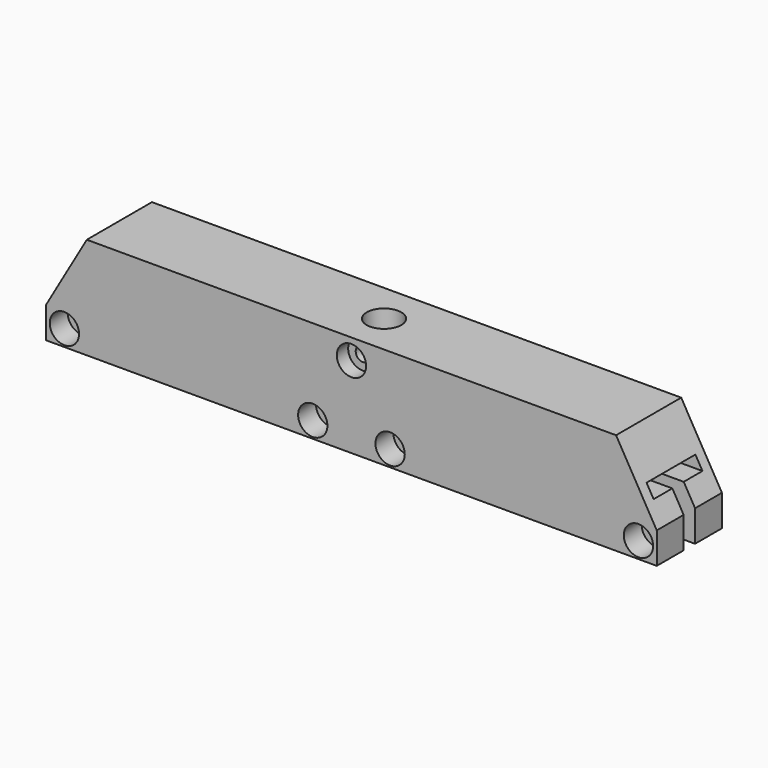
from build123d import *

# Parameters (mm, degrees)
F1_DEPTH       = 10
F3_DEPTH       = 7.5
F5_R           = 4.25
F6_DEPTH       = 30
F8_D           = 4
F8_DEPTH       = 8.5
F8_CBORE_D     = 7.2
F8_CBORE_DEPTH = 5.5
F8_TIP         = 1.2017212381
F9_D           = 3.5
F9_DEPTH       = 7
F9_CBORE_D     = 7.2
F9_CBORE_DEPTH = 3.5
F9_TIP         = 1.0515060833
F10_R          = 5
F11_R          = 5
F12_W          = 3.5
F12_H          = 12.5
F13_DEPTH      = 150.001
F7_R           = 1.1
F14_DEPTH      = 18
F15_T1_DEPTH   = 109.6192794117
F16_T1_DEPTH   = 109.6192794117


# Not quite as in the source:
# - a fillet or chamfer that OpenCascade refuses, or shapes differently, is made with other operations: its cross-section is extruded or revolved along the edge and cut away or added


with BuildPart() as f1:
    # F0 (on Front) → F1 (new body)
    with BuildSketch(Plane.XZ):
        Polygon((75, 12.5), (-75, 12.5), (-75, -12.5), (-50.5, -12.5), (75, -12.5), align=None)
    extrude(amount=-F1_DEPTH)

    # F2 (on face) → F3 (cut)
    with BuildSketch(Plane.XZ):
        with BuildLine():
            Line((-50.5, 0), (-50.5, -12.5))
            Line((-50.5, -12.5), (-29.5, -12.5))
            Line((-29.5, -12.5), (-29.5, 0))
            ThreePointArc((-29.5, 0), (-29.5018489924, 1.0611519764), (-29.616133488, 2.116133488))
            ThreePointArc((-29.616133488, 2.116133488), (-32.4157560185, 7.5842439815), (-37.883866512, 10.383866512))
            ThreePointArc((-37.883866512, 10.383866512), (-38.9388480236, 10.4981510076), (-40, 10.5))
            ThreePointArc((-40, 10.5), (-46.7951402173, 8.2937242033), (-50.383866512, 2.116133488))
            ThreePointArc((-50.383866512, 2.116133488), (-50.4981510076, 1.0611519764), (-50.5, 0))
        make_face()
        with BuildLine():
            ThreePointArc((29.616133488, 2.116133488), (29.5018489924, 1.0611519764), (29.5, 0))
            Line((29.5, 0), (29.5, -12.5))
            Line((29.5, -12.5), (50.5, -12.5))
            Line((50.5, -12.5), (50.5, 0))
            ThreePointArc((50.5, 0), (50.4981510076, 1.0611519764), (50.383866512, 2.116133488))
            ThreePointArc((50.383866512, 2.116133488), (47.5842439815, 7.5842439815), (42.116133488, 10.383866512))
            ThreePointArc((42.116133488, 10.383866512), (41.0611519764, 10.4981510076), (40, 10.5))
            ThreePointArc((40, 10.5), (38.9388480236, 10.4981510076), (37.883866512, 10.383866512))
            ThreePointArc((37.883866512, 10.383866512), (32.4157560185, 7.5842439815), (29.616133488, 2.116133488))
        make_face()
        with BuildLine():
            Line((-65, -12.5), (-59.4149563834, -12.5))
            Line((-59.4149563834, -12.5), (-50.5, -12.5))
            Line((-50.5, -12.5), (-50.5, 0))
            ThreePointArc((-50.5, 0), (-50.4981510076, 1.0611519764), (-50.383866512, 2.116133488))
            Line((-50.383866512, 2.116133488), (-65, -12.5))
        make_face()
        Polygon((-29.5, 0), (-29.5, -12.5), (-15, -12.5), (-27.5, 0), align=None)
        with BuildLine():
            ThreePointArc((-29.616133488, 2.116133488), (-29.5018489924, 1.0611519764), (-29.5, 0))
            Line((-29.5, 0), (-27.5, 0))
            Line((-27.5, 0), (-29.616133488, 2.116133488))
        make_face()
        Polygon((27.5, 0), (15, -12.5), (17, -12.5), (19.8756534234, -12.5), (29.5, -12.5), (29.5, 0), align=None)
        with BuildLine():
            Line((29.616133488, 2.116133488), (27.5, 0))
            Line((27.5, 0), (29.5, 0))
            ThreePointArc((29.5, 0), (29.5018489924, 1.0611519764), (29.616133488, 2.116133488))
        make_face()
        with BuildLine():
            Line((50.5, 0), (52.5, 0))
            Line((52.5, 0), (50.383866512, 2.116133488))
            ThreePointArc((50.383866512, 2.116133488), (50.4981510076, 1.0611519764), (50.5, 0))
        make_face()
        Polygon((62.5, -10.8300764114), (62.5, -10), (52.5, 0), (50.5, 0), (50.5, -12.5), (62.5, -12.5), align=None)
        Polygon((62.5, -12.5), (65, -12.5), (62.5, -10), (62.5, -10.8300764114), align=None)
    extrude(amount=-F3_DEPTH, mode=Mode.SUBTRACT)

    # F4: F1 across face


with BuildPart() as f1_1:
    add(f1.part)
    add(f1.part.mirror(Plane.XZ))

    # F5 (on face) → F6 (cut)
    with BuildSketch(Plane.XY.offset(12.5)):
        Circle(F5_R)
    extrude(amount=-F6_DEPTH, mode=Mode.SUBTRACT)

    # F8
    with Locations(Plane.XZ.offset(10)):
        with Locations((-70.5, -8.5), (-9.5, -8.5), (9.5, -8.5), (70.5, -8.5)):
            CounterBoreHole(F8_D / 2, F8_CBORE_D / 2, F8_CBORE_DEPTH, depth=F8_DEPTH)
            with Locations((0, 0, -(F8_DEPTH + F8_TIP / 2))):  # 118° drill point
                Cone(0, F8_D / 2, F8_TIP, mode=Mode.SUBTRACT)

    # F9
    with Locations(Plane.XZ.offset(10)):
        with Locations((0, 7.5)):
            CounterBoreHole(F9_D / 2, F9_CBORE_D / 2, F9_CBORE_DEPTH, depth=F9_DEPTH)
            with Locations((0, 0, -(F9_DEPTH + F9_TIP / 2))):  # 118° drill point
                Cone(0, F9_D / 2, F9_TIP, mode=Mode.SUBTRACT)

    # F10
    f10_edges = [f1_1.edges().sort_by_distance(p)[0] for p in [
        (-29.616133, 0, 2.116133),
    ]]
    fillet(f10_edges, radius=F10_R)

    # F11
    f11_edges = [f1_1.edges().sort_by_distance(p)[0] for p in [
        (-50.383867, 0, 2.116133),
    ]]
    fillet(f11_edges, radius=F11_R)

    # F12 (on face) → F13 (cut, through all)
    with BuildSketch(Plane.YZ.offset(75)):
        with Locations((0, -6.25)):
            Rectangle(F12_W, F12_H)
        Polygon((-7.5, 0), (-1.75, 0), (1.75, 0), (7.5, 0), (7.5, 3), (-7.5, 3), align=None)
    extrude(amount=-F13_DEPTH, mode=Mode.SUBTRACT)

    # F7 (on face) → F14 (cut)
    with BuildSketch(Plane.XZ.offset(10)):
        with Locations((-70.5, -8.5)):
            Circle(F7_R)
        with Locations((-9.5, -8.5)):
            Circle(F7_R)
        with Locations((9.5, -8.5)):
            Circle(F7_R)
        with Locations((70.5, -8.5)):
            Circle(F7_R)
    extrude(amount=-F14_DEPTH, mode=Mode.SUBTRACT)

    # F15: chamfer of 10 x 17.3205080757 on 1 edges, made by hand

    # F15_s2 → F15_t1 (cut)
    with BuildSketch(Plane.XZ.offset(-54.8096397058)):
        Polygon((-75, -4.8205080757), (-65, 12.5), (-75, 12.5), align=None)
    extrude(amount=F15_T1_DEPTH, mode=Mode.SUBTRACT)

    # F16: chamfer of 10 x 17.3205080757 on 1 edges, made by hand

    # F16_s2 → F16_t1 (cut)
    with BuildSketch(Plane.XZ.offset(-54.8096397058)):
        Polygon((75, -4.8205080757), (65, 12.5), (75, 12.5), align=None)
    extrude(amount=F16_T1_DEPTH, mode=Mode.SUBTRACT)


solid = f1_1.part
